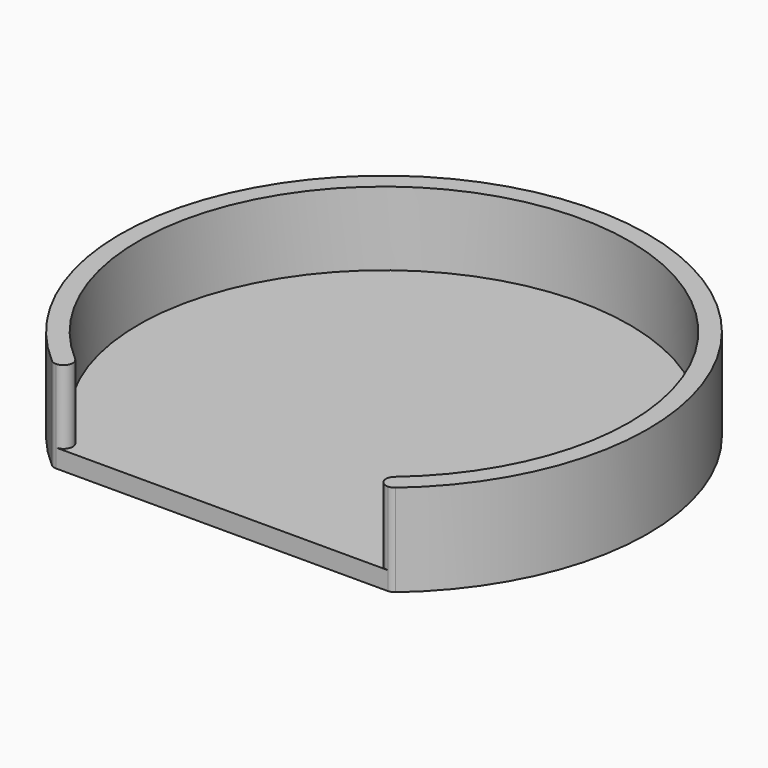
from build123d import *

# Parameters (mm, degrees)
F1_DEPTH = 15
F2_DEPTH = 3
F3_R     = 1.49999


# Not quite as in the source:
# - a fillet or chamfer is up to 0.001 mm smaller than in the source, because OpenCascade refuses the exact size


with BuildPart() as f1:
    # F0 (on Top) → F1 (new body)
    with BuildSketch(Plane.XY):
        with BuildLine():
            ThreePointArc((-22.6053091109, -33), (-18.6519119069, 35.3851124376), (40, 0))
            ThreePointArc((40, 0), (35.3851124376, -18.6519119069), (22.6053091109, -33))
            Line((22.6053091109, -33), (27.5680975042, -33))
            ThreePointArc((27.5680975042, -33), (38.9514325326, -18.2149911792), (43, 0))
            ThreePointArc((43, 0), (-18.2149911792, 38.9514325326), (-27.5680975042, -33))
            Line((-27.5680975042, -33), (-22.6053091109, -33))
        make_face()
    extrude(amount=F1_DEPTH)

    # F0 (on Top) → F2 (join)
    with BuildSketch(Plane.XY):
        with BuildLine():
            ThreePointArc((22.6053091109, -33), (35.3851124376, -18.6519119069), (40, 0))
            ThreePointArc((40, 0), (-18.6519119069, 35.3851124376), (-22.6053091109, -33))
            Line((-22.6053091109, -33), (22.6053091109, -33))
        make_face()
    extrude(amount=F2_DEPTH)

    # F3 (radius 1.5 in the source; OpenCascade refuses exactly that, so slightly less here)
    f3_edges = [f1.edges().sort_by_distance(p)[0] for p in [
        (-22.605309, -33, 9),
        (22.605309, -33, 9),
        (-27.568098, -33, 7.5),
        (27.568098, -33, 7.5),
    ]]
    fillet(f3_edges, radius=F3_R)


solid = f1.part
